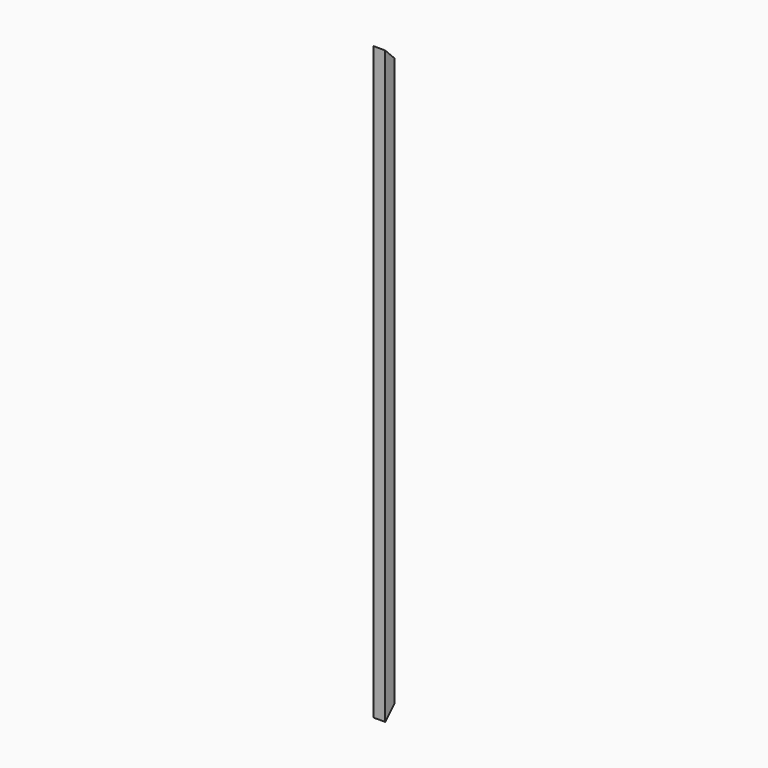
from build123d import *

# Parameters (mm, degrees)
F1_DEPTH   = 504
F2_C1_SIZE = 9.9999
F2_C2_SIZE = 9.9999


# Not quite as in the source:
# - a fillet or chamfer is up to 0.001 mm smaller than in the source, because OpenCascade refuses the exact size


with BuildPart() as f1:
    # F0 (on Top) → F1 (new body)
    with BuildSketch(Plane.XY):
        Polygon((-3, 5), (-5, 5), (-5, -5), (5, -5), (5, 5), (3, 5), (3, -3), (-3, -3), align=None)
    extrude(amount=F1_DEPTH)

    # F2: chamfer of 10 on 4 edges, made by hand

    # F2_c1 (size 10 in the source; OpenCascade refuses exactly that, so slightly less here)
    f2_c1_edges = [f1.edges().sort_by_distance(p)[0] for p in [
        (-4, 5, 0),
    ]]
    chamfer(f2_c1_edges, length=F2_C1_SIZE)

    # F2_c2 (size 10 in the source; OpenCascade refuses exactly that, so slightly less here)
    f2_c2_edges = [f1.edges().sort_by_distance(p)[0] for p in [
        (-4, 5, 504),
    ]]
    chamfer(f2_c2_edges, length=F2_C2_SIZE)


solid = f1.part
